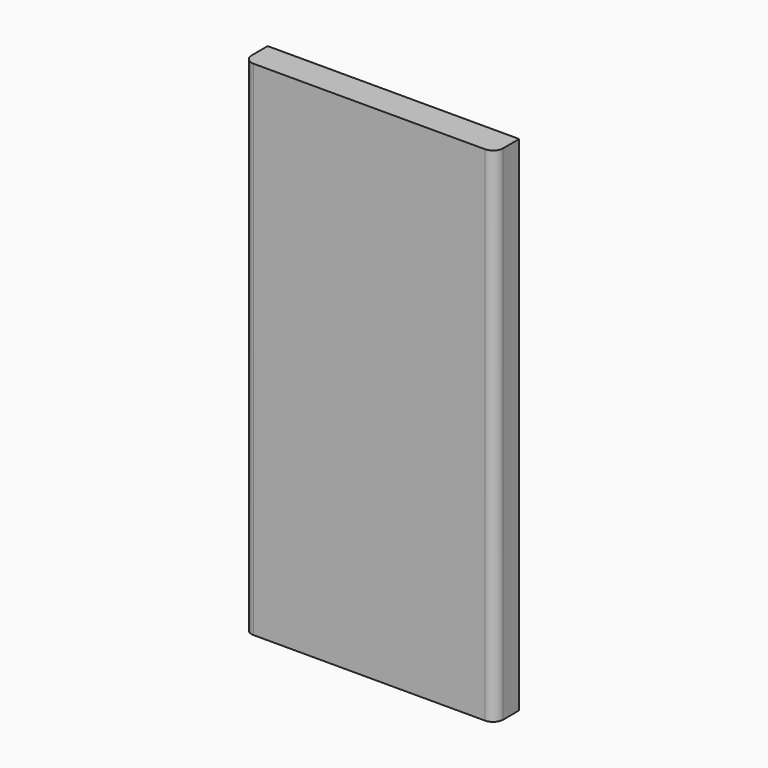
from build123d import *

# Parameters (mm, degrees)
F0_W     = 25
F0_H     = 50
F1_DEPTH = 3
F2_R     = 1


with BuildPart() as f1:
    # F0 (on Front) → F1 (new body)
    with BuildSketch(Plane.XZ):
        with Locations((-11.1966824625, -9.4222032943)):
            Rectangle(F0_W, F0_H)
    extrude(amount=F1_DEPTH)

    # F2
    f2_edges = [f1.edges().sort_by_distance(p)[0] for p in [
        (-23.696682, -3, -9.422203),
        (1.303318, -3, -9.422203),
    ]]
    fillet(f2_edges, radius=F2_R)


solid = f1.part
